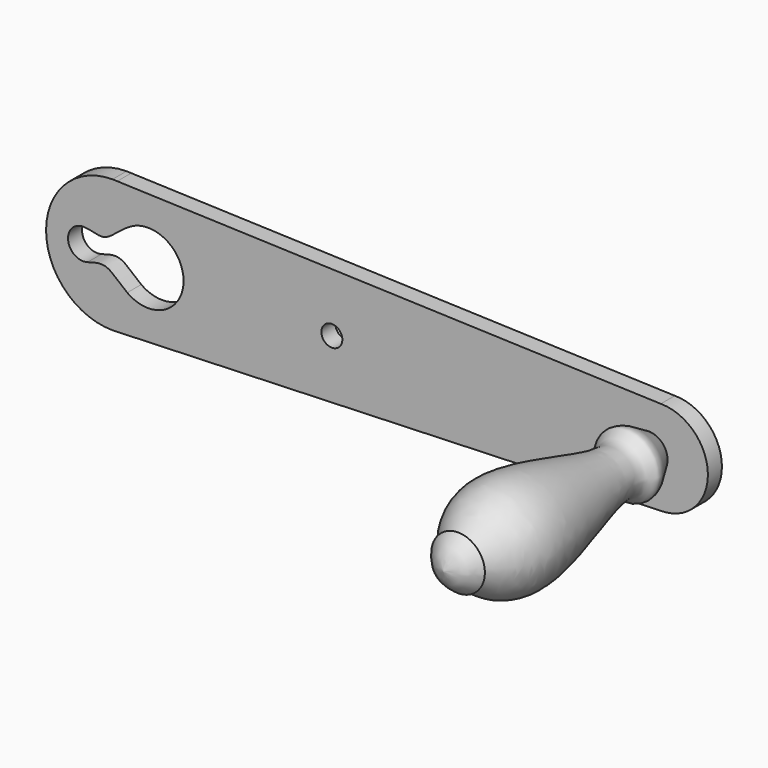
from build123d import *

# Parameters (mm, degrees)
F1_DEPTH = 2.3
F2_R     = 1.375
F3_DEPTH = 2.3
F2_R_2   = 2.49
F4_DEPTH = 31.27


# Not quite as in the source:
# - a feature names something its author has since deleted; it is built from what else it names


with BuildPart() as f1:
    # F0 (on Front) → F1 (new body)
    with BuildSketch(Plane.XZ):
        with BuildLine():
            Line((-40.9890707389, 8.72), (-40.3740798098, 8.698286392))
            ThreePointArc((-40.3740798098, 8.698286392), (-40.6813836724, 8.7145699073), (-40.9890707389, 8.72))
        make_face()
        with BuildLine():
            Line((30.9509292611, 6.18), (-40.3740798098, 8.698286392))
            Line((-40.3740798098, 8.698286392), (-40.9890707389, 8.72))
            ThreePointArc((-40.9890707389, 8.72), (-49.7090707389, 0), (-40.9890707389, -8.72))
            Line((-40.9890707389, -8.72), (-40.3740798098, -8.698286392))
            Line((-40.3740798098, -8.698286392), (30.9509292611, -6.18))
            ThreePointArc((30.9509292611, -6.18), (37.1309292611, 0), (30.9509292611, 6.18))
        make_face()
        with BuildLine():
            Line((-40.3740798098, -8.698286392), (-40.9890707389, -8.72))
            ThreePointArc((-40.9890707389, -8.72), (-40.6813836724, -8.7145699073), (-40.3740798098, -8.698286392))
        make_face()
    extrude(amount=F1_DEPTH)

    # F2 (on face) → F3 (cut, through all)
    with BuildSketch(Plane.XZ.offset(2.3)):
        with BuildLine():
            ThreePointArc((-31.6690707389, 0), (-33.9402317237, 3.9926073348), (-38.5327578563, 4.0808641824))
            ThreePointArc((-38.5327578563, 4.0808641824), (-40.9486127259, 0.3115213811), (-39.0589409979, -3.7472272764))
            ThreePointArc((-39.0589409979, -3.7472272764), (-34.2133443589, -4.142821946), (-31.6690707389, 0))
        make_face()
        with BuildLine():
            ThreePointArc((-44.2763140533, -1.9220978244), (-43.231335878, -1.2030142619), (-42.8290707389, 0))
            ThreePointArc((-42.8290707389, 0), (-43.3830840877, 1.3817100291), (-44.7381933434, 1.9979342579))
            ThreePointArc((-44.7381933434, 1.9979342579), (-46.8153308148, -0.2340318586), (-44.2763140533, -1.9220978244))
        make_face()
        with BuildLine():
            ThreePointArc((-44.7381933434, 1.9979342579), (-43.3830840877, 1.3817100291), (-42.8290707389, 0))
            ThreePointArc((-42.8290707389, 0), (-43.231335878, -1.2030142619), (-44.2763140533, -1.9220978244))
            add(Edge.make_bspline(
                [(-44.2763140533, -1.9220978244), (-43.4539093283, -1.685590762), (-41.685646855, -1.0885271587), (-40.1825261621, -2.924193264), (-39.0589409979, -3.7472272764)],
                knots=[0, 0, 0, 0, 0.4500424394, 1, 1, 1, 1], degree=3))
            ThreePointArc((-39.0589409979, -3.7472272764), (-40.9486127259, 0.3115213811), (-38.5327578563, 4.0808641824))
            add(Edge.make_bspline(
                [(-44.7381933434, 1.9979342579), (-43.6566289581, 1.9487385679), (-41.8853510694, 0.927471279), (-40.0561887145, 3.2526042187), (-38.5327578563, 4.0808641824)],
                knots=[0, 0, 0, 0, 0.4416856432, 1, 1, 1, 1], degree=3))
        make_face()
        with Locations((-12.2090707389, 0)):
            Circle(F2_R)
    extrude(amount=-F3_DEPTH, mode=Mode.SUBTRACT)

    # F2 (on face) → F4 (join)
    with BuildSketch(Plane.XZ.offset(2.3)):
        with Locations((29.3509292611, 0)):
            Circle(F2_R_2)
    extrude(amount=F4_DEPTH)

    # F5 (on Top) → F7 (revolve)
    with BuildSketch(Plane.XY):
        with BuildLine():
            add(Edge.make_bspline(
                [(29.3601173908, -35.9721258283), (30.1185949648, -35.7541623267), (31.6059828087, -35.326732072), (32.45773849, -34.1395743071), (32.8751504421, -33.5577949882)],
                knots=[0, 0, 0, 0, 0.509939339, 1, 1, 1, 1], degree=3))
            Line((32.8751504421, -33.5577949882), (29.3601173908, -33.570792526))
            Line((29.3601173908, -33.570792526), (29.3601173908, -35.9721258283))
        make_face()
    revolve(axis=Axis((29.3601173908, -17.865916132, 0), (0, -1, 0)))


with BuildPart() as f6:
    # F5 (on Top) → F6 (revolve)
    with BuildSketch(Plane.XY):
        with BuildLine():
            add(Edge.make_bspline(
                [(31.8413078785, -2.3), (32.7217720858, -3.7490035606), (34.4577278681, -6.1824333871), (30.5829934083, -7.2105587452), (38.8755879035, -26.4733960087), (33.8892173922, -31.5047864924), (31.8413078785, -33.5577949882)],
                knots=[0, 0, 0, 0, 0.1881491817, 0.3167473972, 0.7168077329, 1, 1, 1, 1], degree=3))
            Line((31.8413078785, -2.3), (31.8413078785, -33.5577949882))
        make_face()
    revolve(axis=Axis((29.3601173908, -17.865916132, 0), (0, -1, 0)))


solid = Compound([f1.part, f6.part])
